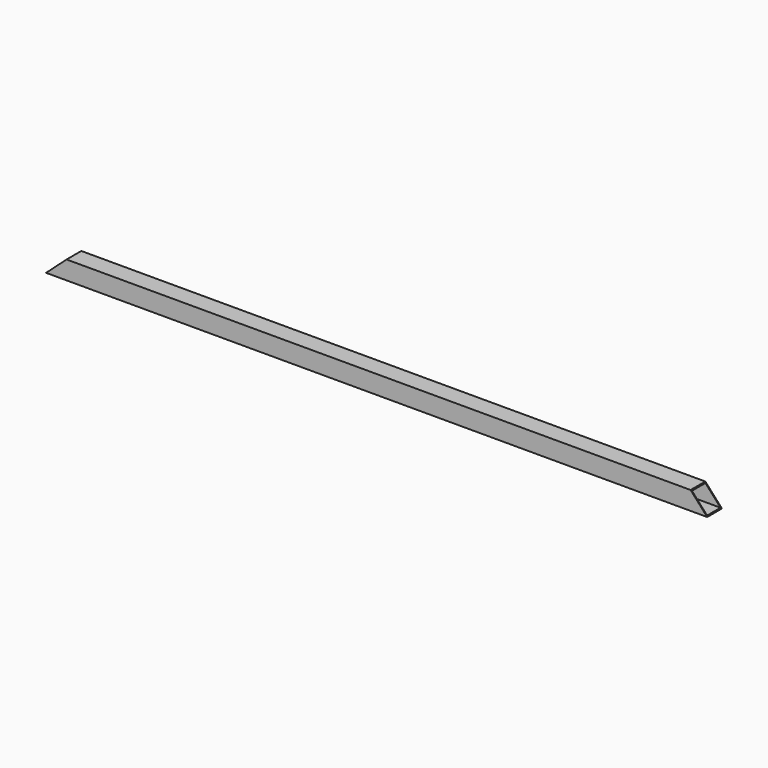
from build123d import *

# Parameters (mm, degrees)
F0_W          = 1366.8883
F0_H          = 38.1
F1_DEPTH      = 38.1
F2_W          = 34.798
F2_H          = 34.798
F3_DEPTH      = 683.44515
F3_DEPTH_BACK = 683.44515
F5_DEPTH      = 38.101


# Not quite as in the source:
# - a feature names something its author has since deleted; it is built from what else it names


with BuildPart() as f1:
    # F0 (on Front) → F1 (new body)
    with BuildSketch(Plane.XZ):
        with Locations((0, -19.05)):
            Rectangle(F0_W, F0_H)
    extrude(amount=F1_DEPTH)

    # F2 (on Right) → F3 (cut, two sides)
    with BuildSketch(Plane.YZ) as f3_sk:
        with Locations((-19.05, -19.05)):
            Rectangle(F2_W, F2_H)
    extrude(amount=-F3_DEPTH, mode=Mode.SUBTRACT)
    extrude(f3_sk.sketch, amount=F3_DEPTH_BACK, mode=Mode.SUBTRACT)

    # F4 (on face) → F5 (cut, through all)
    with BuildSketch(Plane.XZ.offset(38.1)):
        Polygon((649.1544057584, 0), (683.44415, -38.1), (683.44415, 0), align=None)
        Polygon((-683.44415, 0), (-683.44415, -38.1), (-641.1108166729, 0), align=None)
    extrude(amount=-F5_DEPTH, mode=Mode.SUBTRACT)


solid = f1.part
